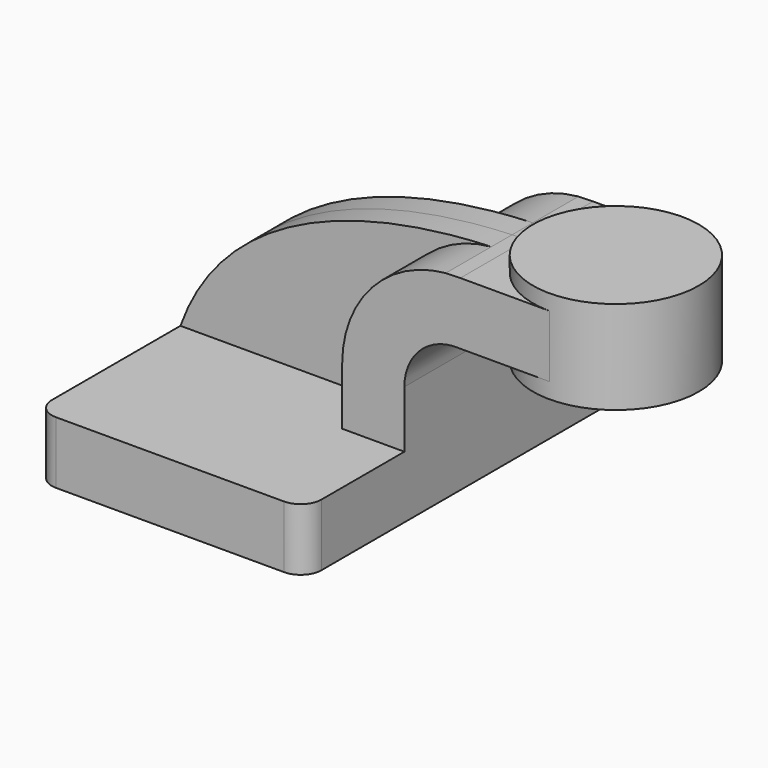
from build123d import *

# Parameters (mm, degrees)
F1_DEPTH = 63.5
F2_DEPTH = 25.4
F3_DEPTH = 7.9375
F4_DEPTH = 25.4
F0_W     = 25.4
F0_H     = 4.7498
F0_H_2   = 4.7752
F6_R     = 6.35


with BuildPart() as f1:
    # F0 (on Front) → F1 (new body, symmetric)
    with BuildSketch(Plane.XZ):
        Polygon((22.225, 9.525), (-41.275, 9.525), (-41.275, -9.525), (41.275, -9.525), (41.275, 9.525), align=None)
    extrude(amount=F1_DEPTH, both=True)

    # F0 (on Front) → F2 (join, symmetric)
    with BuildSketch(Plane.XZ):
        with BuildLine():
            Line((22.225, 27.0233751515), (22.225, 9.525))
            Line((22.225, 9.525), (41.275, 9.525))
            Line((41.275, 9.525), (41.275, 27.0233751515))
            ThreePointArc((41.275, 27.0233751515), (46.232053506, 38.5478738111), (58.0074811786, 42.8752))
            Line((58.0074811786, 42.8752), (60.325, 42.8752))
            Line((60.325, 42.8752), (60.325, 61.9252))
            Line((60.325, 61.9252), (58.4221034718, 61.9252))
            add(Edge.make_bspline(
                [(53.9455429382, 61.8010559243), (55.4372337649, 61.858340914), (56.9298403376, 61.8995627303), (58.4221034718, 61.9252)],
                knots=[108.7173325618, 108.7173325618, 108.7173325618, 108.7173325618, 112.6290078119, 112.6290078119, 112.6290078119, 112.6290078119], degree=3))
            ThreePointArc((53.9455429382, 61.8010559243), (31.3462087293, 50.5588798425), (22.225, 27.0233751515))
        make_face()
    extrude(amount=F2_DEPTH, both=True)

    # F0 (on Front) → F3 (join, symmetric)
    with BuildSketch(Plane.XZ):
        with BuildLine():
            add(Edge.make_bspline(
                [(-41.275, 9.525), (-28.2643212455, 46.2087638667), (12.486925514, 60.2089321217), (53.9455429382, 61.8010559243)],
                knots=[0, 0, 0, 0, 108.7173325618, 108.7173325618, 108.7173325618, 108.7173325618], degree=3))
            Line((-41.275, 9.525), (22.225, 9.525))
            Line((22.225, 9.525), (22.225, 27.0233751515))
            ThreePointArc((22.225, 27.0233751515), (31.3462087293, 50.5588798425), (53.9455429382, 61.8010559243))
        make_face()
    extrude(amount=F3_DEPTH, both=True)

    # F4 (add): a face of the model
    f4_faces = [f1.faces().sort_by_distance(p)[0] for p in [
        (60.325, 0, 52.4002),
    ]]
    extrude(f4_faces, amount=F4_DEPTH)

    # F0 (on Front) → F5 (revolve)
    with BuildSketch(Plane.XZ):
        with Locations((98.425, 64.3001)):
            Rectangle(F0_W, F0_H)
        Polygon((111.125, 61.9252), (85.725, 61.9252), (85.725, 52.3875), (85.725, 42.8752), (111.125, 42.8752), align=None)
        with Locations((98.425, 40.4876)):
            Rectangle(F0_W, F0_H_2)
    revolve(axis=Axis((85.725, 0, 52.3875), (0, 0, 1)))

    # F6
    f6_edges = [f1.edges().sort_by_distance(p)[0] for p in [
        (41.275, -63.5, 0),
        (-41.275, -63.5, 0),
        (41.275, 63.5, 0),
        (-41.275, 63.5, 0),
    ]]
    fillet(f6_edges, radius=F6_R)


solid = f1.part
